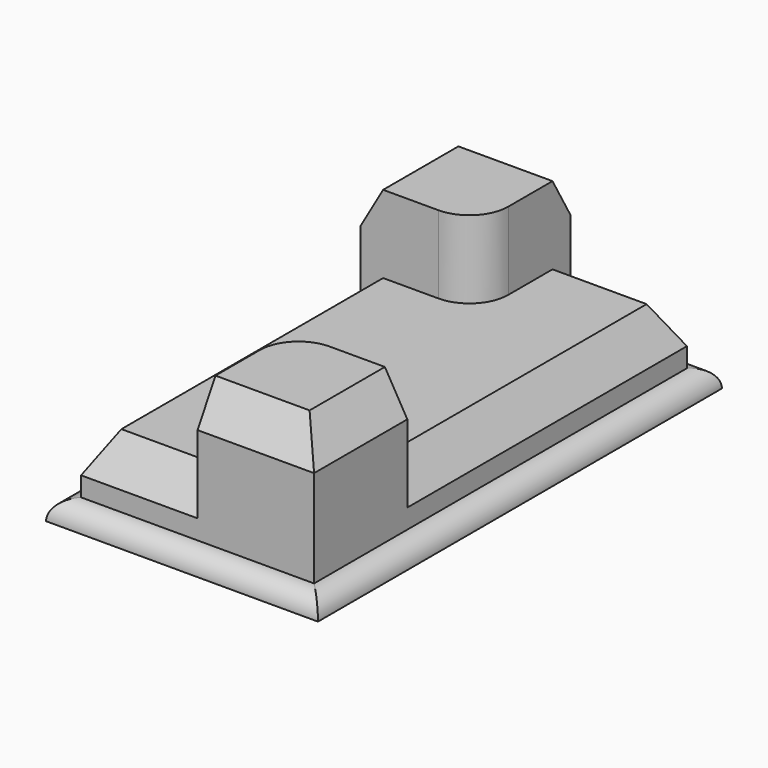
from build123d import *

# Parameters (mm, degrees)
F0_W       = 88.9
F0_H       = 165.1
F1_DEPTH   = 6.35
F2_DEPTH   = 25.4
F3_DEPTH   = 50.8
F4_SIZE2   = 12.7
F4_SIZE    = 7.3323484187
F4_2_SIZE2 = 12.7
F4_2_SIZE  = 7.3323484187
F4_3_SIZE2 = 12.7
F4_3_SIZE  = 7.3323484187
F5_R       = 6.34999


# Not quite as in the source:
# - a fillet or chamfer is up to 0.001 mm smaller than in the source, because OpenCascade refuses the exact size


with BuildPart() as f1:
    # F0 (on Top) → F1 (new body)
    with BuildSketch(Plane.XY):
        with Locations((0, -76.2)):
            Rectangle(F0_W, F0_H)
        Polygon((-38.1, -38.1), (-38.1, 0), (0, 0), (38.1, 0), (38.1, -114.3), (38.1, -152.4), (0, -152.4), (-38.1, -152.4), align=None, mode=Mode.SUBTRACT)
        with BuildLine():
            Line((-12.7, -38.1), (-38.1, -38.1))
            Line((-38.1, -38.1), (-38.1, -152.4))
            Line((-38.1, -152.4), (0, -152.4))
            Line((0, -152.4), (0, -127))
            ThreePointArc((0, -127), (3.7197438789, -118.0197438789), (12.7, -114.3))
            Line((12.7, -114.3), (38.1, -114.3))
            Line((38.1, -114.3), (38.1, 0))
            Line((38.1, 0), (0, 0))
            Line((0, 0), (0, -25.4))
            ThreePointArc((0, -25.4), (-3.7197438789, -34.3802561211), (-12.7, -38.1))
        make_face()
        with BuildLine():
            Line((0, 0), (-38.1, 0))
            Line((-38.1, 0), (-38.1, -38.1))
            Line((-38.1, -38.1), (-12.7, -38.1))
            ThreePointArc((-12.7, -38.1), (-3.7197438789, -34.3802561211), (0, -25.4))
            Line((0, -25.4), (0, 0))
        make_face()
        with BuildLine():
            Line((0, -127), (0, -152.4))
            Line((0, -152.4), (38.1, -152.4))
            Line((38.1, -152.4), (38.1, -114.3))
            Line((38.1, -114.3), (12.7, -114.3))
            ThreePointArc((12.7, -114.3), (3.7197438789, -118.0197438789), (0, -127))
        make_face()
    extrude(amount=F1_DEPTH)

    # F0 (on Top) → F2 (join)
    with BuildSketch(Plane.XY):
        with BuildLine():
            Line((-12.7, -38.1), (-38.1, -38.1))
            Line((-38.1, -38.1), (-38.1, -152.4))
            Line((-38.1, -152.4), (0, -152.4))
            Line((0, -152.4), (0, -127))
            ThreePointArc((0, -127), (3.7197438789, -118.0197438789), (12.7, -114.3))
            Line((12.7, -114.3), (38.1, -114.3))
            Line((38.1, -114.3), (38.1, 0))
            Line((38.1, 0), (0, 0))
            Line((0, 0), (0, -25.4))
            ThreePointArc((0, -25.4), (-3.7197438789, -34.3802561211), (-12.7, -38.1))
        make_face()
    extrude(amount=F2_DEPTH)

    # F0 (on Top) → F3 (join)
    with BuildSketch(Plane.XY):
        with BuildLine():
            Line((0, -127), (0, -152.4))
            Line((0, -152.4), (38.1, -152.4))
            Line((38.1, -152.4), (38.1, -114.3))
            Line((38.1, -114.3), (12.7, -114.3))
            ThreePointArc((12.7, -114.3), (3.7197438789, -118.0197438789), (0, -127))
        make_face()
        with BuildLine():
            Line((0, 0), (-38.1, 0))
            Line((-38.1, 0), (-38.1, -38.1))
            Line((-38.1, -38.1), (-12.7, -38.1))
            ThreePointArc((-12.7, -38.1), (-3.7197438789, -34.3802561211), (0, -25.4))
            Line((0, -25.4), (0, 0))
        make_face()
    extrude(amount=F3_DEPTH)

    # F4
    f4_edges = [f1.edges().sort_by_distance(p)[0] for p in [
        (-38.1, -95.25, 25.4),
        (-19.05, -152.4, 25.4),
        (38.1, -57.15, 25.4),
        (19.05, 0, 25.4),
    ]]
    f4_side = f1.faces().sort_by_distance((0, -76.2, 25.4))[0]
    chamfer(f4_edges, length=F4_SIZE, length2=F4_SIZE2, reference=f4_side)

    # F4#2
    f4_2_edges = [f1.edges().sort_by_distance(p)[0] for p in [
        (38.1, -133.35, 50.8),
        (19.05, -152.4, 50.8),
    ]]
    f4_2_side = f1.faces().sort_by_distance((19.446042, -133.746042, 50.8))[0]
    chamfer(f4_2_edges, length=F4_2_SIZE, length2=F4_2_SIZE2, reference=f4_2_side)

    # F4#3
    f4_3_edges = [f1.edges().sort_by_distance(p)[0] for p in [
        (-19.05, 0, 50.8),
        (-38.1, -19.05, 50.8),
    ]]
    f4_3_side = f1.faces().sort_by_distance((-19.446042, -18.653958, 50.8))[0]
    chamfer(f4_3_edges, length=F4_3_SIZE, length2=F4_3_SIZE2, reference=f4_3_side)

    # F5 (radius 6.35 in the source; OpenCascade refuses exactly that, so slightly less here)
    f5_edges = [f1.edges().sort_by_distance(p)[0] for p in [
        (44.45, -76.2, 6.35),
        (0, 6.35, 6.35),
        (-44.45, -76.2, 6.35),
        (0, -158.75, 6.35),
    ]]
    fillet(f5_edges, radius=F5_R)


solid = f1.part
